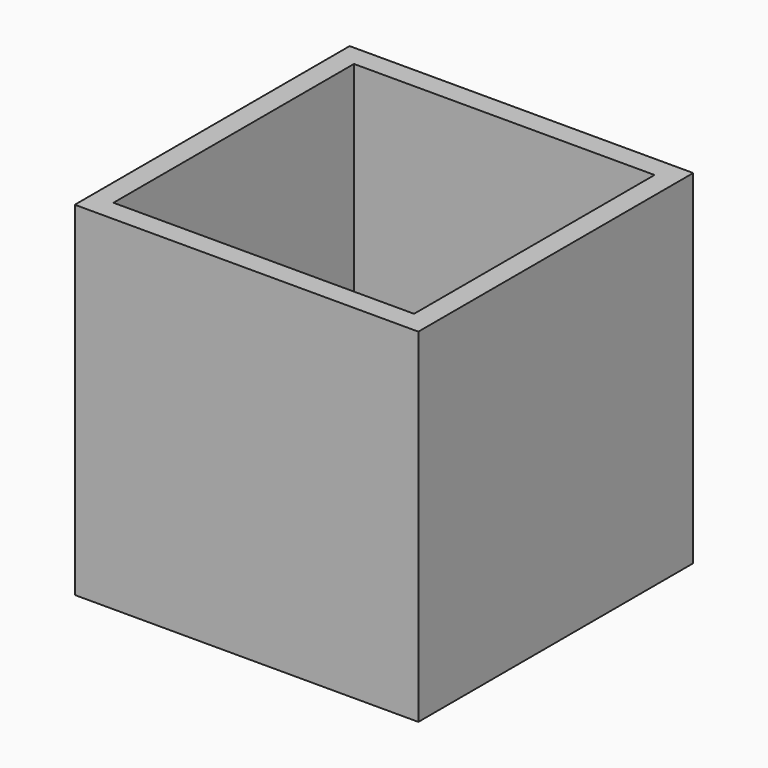
from build123d import *

# Parameters (mm, degrees)
F1_W     = 25.4
F1_H     = 25.4
F1_W_2   = 22.225
F1_H_2   = 22.225
F2_DEPTH = 25.4


# Not quite as in the source:
# - a variable given as a bare number and used for a length is read in inches; the dataset says mm whatever the document's units were


with BuildPart() as f2:
    # F1 (on Top) → F2 (new body)
    with BuildSketch(Plane.XY):
        Rectangle(F1_W, F1_H)
        Rectangle(F1_W_2, F1_H_2, mode=Mode.SUBTRACT)
    extrude(amount=F2_DEPTH)


solid = f2.part
